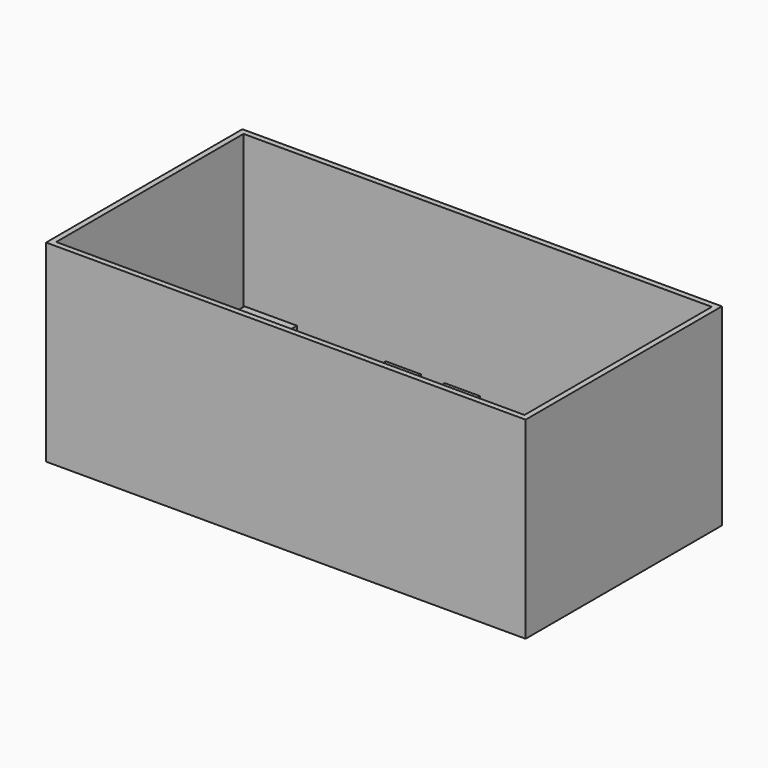
from build123d import *

# Parameters (mm, degrees)
F0_R      = 3
F0_R_2    = 1.375
F1_DEPTH  = 1
F2_W      = 12
F2_H      = 12
F3_DEPTH  = 1
F4_W      = 11.2
F4_H      = 9
F5_DEPTH  = 3.5
F6_W      = 7.5
F6_H      = 4.5
F7_DEPTH  = 2.7
F8_R      = 3
F8_R_2    = 1.375
F9_DEPTH  = 5
F11_ANGLE = 270
F12_W     = 100
F12_H     = 40
F13_DEPTH = 50
F14_T     = 1.2


# Not quite as in the source:
# - a feature names something its author has since deleted; it is built from what else it names


with BuildPart() as f1:
    # F0 (on Top) → F1 (new body)
    with BuildSketch(Plane.XY):
        with BuildLine():
            Line((25.2664580047, 20.9954980612), (-33.7335419953, 20.9954980612))
            ThreePointArc((-33.7335419953, 20.9954980612), (-35.8548623388, 20.1168184047), (-36.7335419953, 17.9954980612))
            Line((-36.7335419953, 17.9954980612), (-36.7335419953, -6.0045019388))
            ThreePointArc((-36.7335419953, -6.0045019388), (-35.8548623388, -8.1258222824), (-33.7335419953, -9.0045019388))
            Line((-33.7335419953, -9.0045019388), (25.2664580047, -9.0045019388))
            ThreePointArc((25.2664580047, -9.0045019388), (27.3877783483, -8.1258222824), (28.2664580047, -6.0045019388))
            Line((28.2664580047, -6.0045019388), (28.2664580047, 17.9954980612))
            ThreePointArc((28.2664580047, 17.9954980612), (27.3877783483, 20.1168184047), (25.2664580047, 20.9954980612))
        make_face()
        with Locations((-33.2335419953, -5.5045019388)):
            Circle(F0_R, mode=Mode.SUBTRACT)
        with Locations((24.7664580047, -5.5045019388)):
            Circle(F0_R, mode=Mode.SUBTRACT)
        with Locations((-33.2335419953, 17.4954980612)):
            Circle(F0_R, mode=Mode.SUBTRACT)
        with Locations((24.7664580047, 17.4954980612)):
            Circle(F0_R, mode=Mode.SUBTRACT)
        with Locations((24.7664580047, -5.5045019388)):
            Circle(F0_R)
        with Locations((24.7664580047, -5.5045019388)):
            Circle(F0_R_2, mode=Mode.SUBTRACT)
        with Locations((24.7664580047, 17.4954980612)):
            Circle(F0_R)
        with Locations((24.7664580047, 17.4954980612)):
            Circle(F0_R_2, mode=Mode.SUBTRACT)
        with Locations((-33.2335419953, -5.5045019388)):
            Circle(F0_R)
        with Locations((-33.2335419953, -5.5045019388)):
            Circle(F0_R_2, mode=Mode.SUBTRACT)
        with Locations((-33.2335419953, 17.4954980612)):
            Circle(F0_R)
        with Locations((-33.2335419953, 17.4954980612)):
            Circle(F0_R_2, mode=Mode.SUBTRACT)
    extrude(amount=-F1_DEPTH)

    # F2 (on face) → F3 (join)
    with BuildSketch(Plane.XY):
        with Locations((-29.7335419953, 7.6954980612)):
            Rectangle(F2_W, F2_H)
    extrude(amount=F3_DEPTH)

    # F4 (on face) → F5 (join)
    with BuildSketch(Plane.XY):
        with Locations((-24.3335419953, -5.1045019388)):
            Rectangle(F4_W, F4_H)
    extrude(amount=F5_DEPTH)

    # F6 (on face) → F7 (join)
    with BuildSketch(Plane.XY):
        with Locations((17.2164580047, -7.3545019388)):
            Rectangle(F6_W, F6_H)
        with Locations((4.6164580047, -7.3545019388)):
            Rectangle(F6_W, F6_H)
    extrude(amount=F7_DEPTH)


with BuildPart() as f9:
    # F8 (on face) → F9 (new body)
    with BuildSketch(Plane(origin=(0, 0, -1), x_dir=(1, 0, 0), z_dir=(0, 0, -1))):
        with Locations((-33.2335419953, 5.5041852891)):
            Circle(F8_R)
        with Locations((-33.2335419953, 5.5041852891)):
            Circle(F8_R_2, mode=Mode.SUBTRACT)
    extrude(amount=F9_DEPTH)


with BuildPart() as f9b:
    # F8 (on face) → F9, piece 2 (new body)
    with BuildSketch(Plane(origin=(0, 0, -1), x_dir=(1, 0, 0), z_dir=(0, 0, -1))):
        with Locations((-33.2335419953, -17.4954980612)):
            Circle(F8_R)
        with Locations((-33.2335419953, -17.4954980612)):
            Circle(F8_R_2, mode=Mode.SUBTRACT)
    extrude(amount=F9_DEPTH)


with BuildPart() as f9c:
    # F8 (on face) → F9, piece 3 (new body)
    with BuildSketch(Plane(origin=(0, 0, -1), x_dir=(1, 0, 0), z_dir=(0, 0, -1))):
        with Locations((24.7664580047, -17.4954980612)):
            Circle(F8_R)
        with Locations((24.7664580047, -17.4954980612)):
            Circle(F8_R_2, mode=Mode.SUBTRACT)
    extrude(amount=F9_DEPTH)


with BuildPart() as f9d:
    # F8 (on face) → F9, piece 4 (new body)
    with BuildSketch(Plane(origin=(0, 0, -1), x_dir=(1, 0, 0), z_dir=(0, 0, -1))):
        with Locations((24.7664580047, 5.5045019388)):
            Circle(F8_R)
        with Locations((24.7664580047, 5.5045019388)):
            Circle(F8_R_2, mode=Mode.SUBTRACT)
    extrude(amount=F9_DEPTH)


with BuildPart() as f1_1:
    # F11: moved
    add(f1.part.rotate(Axis((-4.2335419953, 20.9954980612, 0), (1, 0, 0)), F11_ANGLE))


with BuildPart() as f9_1:
    # F11: moved
    add(f9.part.rotate(Axis((-4.2335419953, 20.9954980612, 0), (1, 0, 0)), F11_ANGLE))


with BuildPart() as f9d_1:
    # F11: moved
    add(f9d.part.rotate(Axis((-4.2335419953, 20.9954980612, 0), (1, 0, 0)), F11_ANGLE))


with BuildPart() as f9c_1:
    # F11: moved
    add(f9c.part.rotate(Axis((-4.2335419953, 20.9954980612, 0), (1, 0, 0)), F11_ANGLE))


with BuildPart() as f9b_1:
    # F11: moved
    add(f9b.part.rotate(Axis((-4.2335419953, 20.9954980612, 0), (1, 0, 0)), F11_ANGLE))


with BuildPart() as f13:
    # F12 (on face) → F13 (new body)
    with BuildSketch(Plane.XZ.offset(-14.9954980612)):
        with Locations((-12.5514894724, 15.9477609955)):
            Rectangle(F12_W, F12_H)
    extrude(amount=-F13_DEPTH)

    # F14
    f14_openings = [f13.faces().sort_by_distance(p)[0] for p in [
        (-12.551489, 39.995498, 35.947761),
    ]]
    offset(amount=F14_T, openings=f14_openings, kind=Kind.INTERSECTION)


solid = Compound([f1_1.part, f9_1.part, f9d_1.part, f9c_1.part, f9b_1.part, f13.part])
